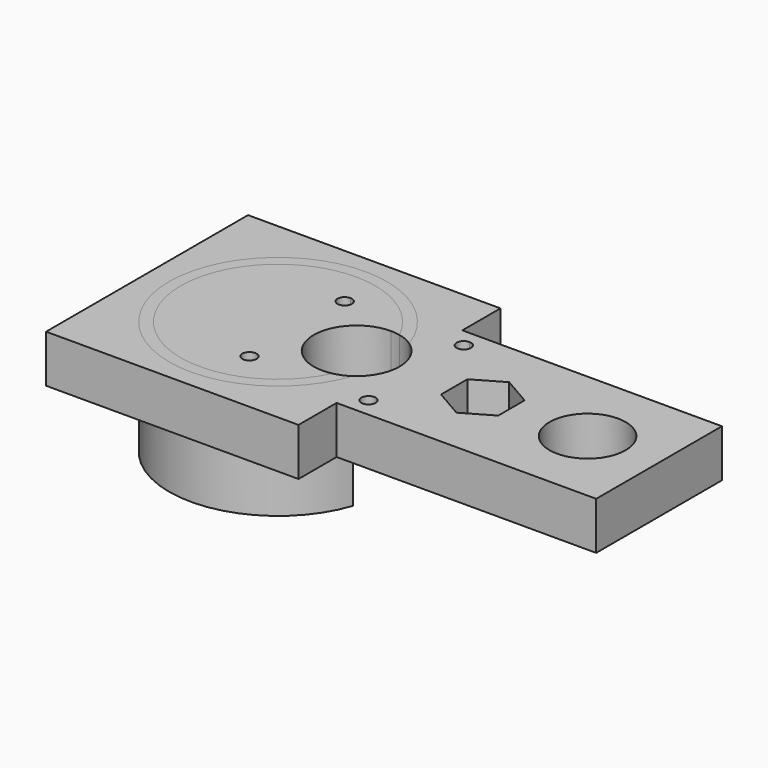
from build123d import *
from build123d import SkipClean  # not in build123d's __all__

# Parameters (mm, degrees)
F0_W      = 101.6
F0_H      = 41.91
F1_DEPTH  = 12.7
F4_DEPTH  = 12.701
F5_R      = 5.08
F6_DEPTH  = 8.636
F7_R      = 10.16
F8_DEPTH  = 12.701
F10_DEPTH = 12.701
F2_R      = 1.905
F12_DEPTH = 25.4
F13_DEPTH = 12.7
F15_DEPTH = 30.48


with BuildPart() as f1:
    # F0 (on Top) → F1 (new body)
    with BuildSketch(Plane.XY):
        with Locations((50.8, 20.955)):
            Rectangle(F0_W, F0_H)
    extrude(amount=F1_DEPTH)

    # F3 (on face) → F4 (cut, through all)
    with BuildSketch(Plane.XY.offset(12.7)):
        with BuildLine():
            ThreePointArc((59.69, 20.955), (58.2021024484, 24.5471024484), (54.61, 26.035))
            ThreePointArc((54.61, 26.035), (51.0178975516, 17.3628975516), (59.69, 20.955))
        make_face()
    extrude(amount=-F4_DEPTH, mode=Mode.SUBTRACT)

    # F5 (on face) → F6 (cut)
    with BuildSketch(Plane.XY.offset(12.7)):
        Polygon((62.23, 16.5555909488), (62.23, 20.955), (62.23, 25.3544090512), (54.61, 29.7538181024), (46.99, 25.3544090512), (46.99, 16.5555909488), (54.61, 12.1561818976), align=None)
        with Locations((54.61, 20.955)):
            Circle(F5_R, mode=Mode.SUBTRACT)
    extrude(amount=-F6_DEPTH, mode=Mode.SUBTRACT)

    # F7 (on face) → F8 (cut, through all)
    with BuildSketch(Plane.XY.offset(12.7)):
        with Locations((82.55, 20.955)):
            Circle(F7_R)
    extrude(amount=-F8_DEPTH, mode=Mode.SUBTRACT)

    # F9 (on face) → F10 (cut, through all)
    with BuildSketch(Plane.XY.offset(12.7)):
        with BuildLine():
            ThreePointArc((20.955, 32.385), (12.872769491, 12.872769491), (32.385, 20.955))
            ThreePointArc((32.385, 20.955), (29.037230509, 29.037230509), (20.955, 32.385))
        make_face()
    extrude(amount=-F10_DEPTH, mode=Mode.SUBTRACT)

    # F2 (on face) → F12 (cut)
    with BuildSketch(Plane.XY.offset(12.7)):
        with BuildLine():
            ThreePointArc((38.735, 36.83), (38.1770384182, 38.1770384182), (36.83, 38.735))
            ThreePointArc((36.83, 38.735), (35.4829615818, 35.4829615818), (38.735, 36.83))
        make_face()
        with Locations((5.08, 5.08)):
            Circle(F2_R)
        with BuildLine():
            ThreePointArc((6.985, 36.83), (6.4270384182, 38.1770384182), (5.08, 38.735))
            ThreePointArc((5.08, 38.735), (3.7329615818, 35.4829615818), (6.985, 36.83))
        make_face()
        with Locations((36.83, 5.08)):
            Circle(F2_R)
    extrude(amount=-F12_DEPTH, mode=Mode.SUBTRACT)

    # F11 (on face) → F13 (join)
    with BuildSketch(Plane.XY.offset(12.7)):
        Polygon((32.385, -12.7), (32.385, 0), (0, 0), (0, 41.91), (32.385, 41.91), (32.385, 54.61), (-34.925, 54.61), (-34.925, -12.7), align=None)
    extrude(amount=-F13_DEPTH)

    # F14 (on face) → F15 (join)
    with BuildSketch(Plane.XY.offset(12.7)):
        with BuildLine():
            ThreePointArc((23.4308703665, 32.1136274213), (25.5340365405, 31.4276942265), (27.4656771106, 30.3494655815))
            ThreePointArc((27.4656771106, 30.3494655815), (-29.0279073084, 20.955), (27.4656771106, 11.5605344185))
            ThreePointArc((27.4656771106, 11.5605344185), (25.5340365405, 10.4823057735), (23.4308703665, 9.7963725787))
            ThreePointArc((23.4308703665, 9.7963725787), (-25.9522764331, 20.955), (23.4308703665, 32.1136274213))
        make_face()
    with SkipClean():  # cleaning this boolean's faces spoils the solid; the shape is the same uncleaned
        extrude(amount=-F15_DEPTH)


solid = f1.part
